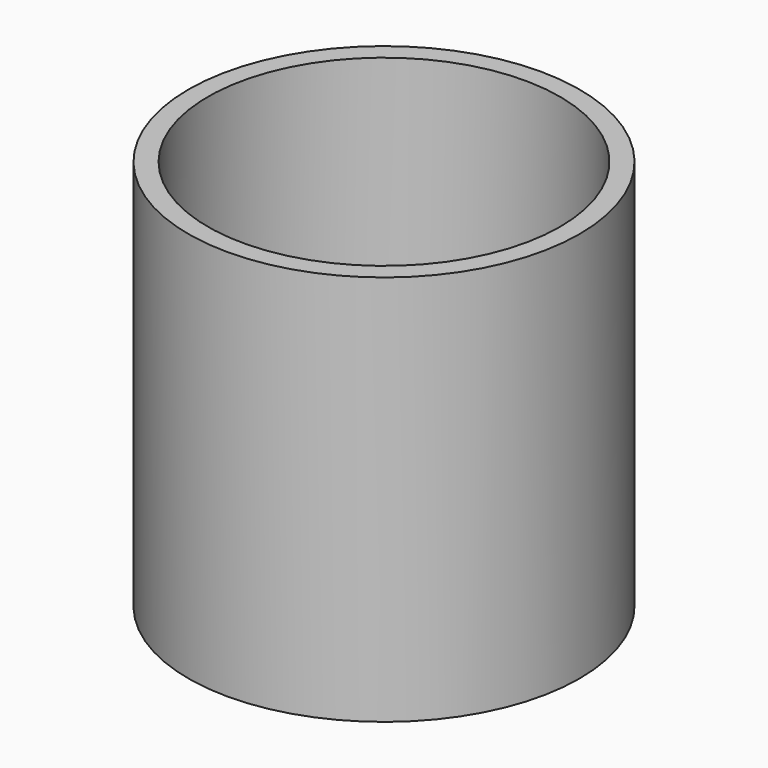
from build123d import *

# Parameters (mm, degrees)
F0_R     = 12.7
F1_DEPTH = 25.4
F2_T     = -1.27
F4_R     = 6.985
F5_DEPTH = 11.43
F7_R     = 1.27


# Not quite as in the source:
# - a fillet or chamfer that OpenCascade refuses, or shapes differently, is made with other operations: its cross-section is extruded or revolved along the edge and cut away or added


with BuildPart() as f1:
    # F0 (on Top) → F1 (new body)
    with BuildSketch(Plane.XY):
        Circle(F0_R)
    extrude(amount=F1_DEPTH)

    # F2
    f2_openings = [f1.faces().sort_by_distance(p)[0] for p in [
        (0, 0, 25.4),
    ]]
    offset(amount=F2_T, openings=f2_openings)

    # F4 (on offset) → F5 (join, through all)
    with BuildSketch(Plane.XY.offset(12.7)):
        Circle(F4_R)
    extrude(amount=-F5_DEPTH)

    # F6: fillet of radius 5.08 on 1 edges, made by hand

    # F6_s1 → F6_t2 (revolve)
    with BuildSketch(Plane.XZ):
        with BuildLine():
            ThreePointArc((11.43, 6.3101562476), (10.16, 2.9500520825), (6.985, 1.27))
            Line((6.985, 1.27), (11.43, 1.27))
            Line((11.43, 1.27), (11.43, 6.3101562476))
        make_face()
    revolve(axis=Axis((0, 0, 1.27), (0, 0, -1)))

    # F7
    f7_edges = [f1.edges().sort_by_distance(p)[0] for p in [
        (-6.985, 0, 1.27),
    ]]
    fillet(f7_edges, radius=F7_R)


solid = f1.part
